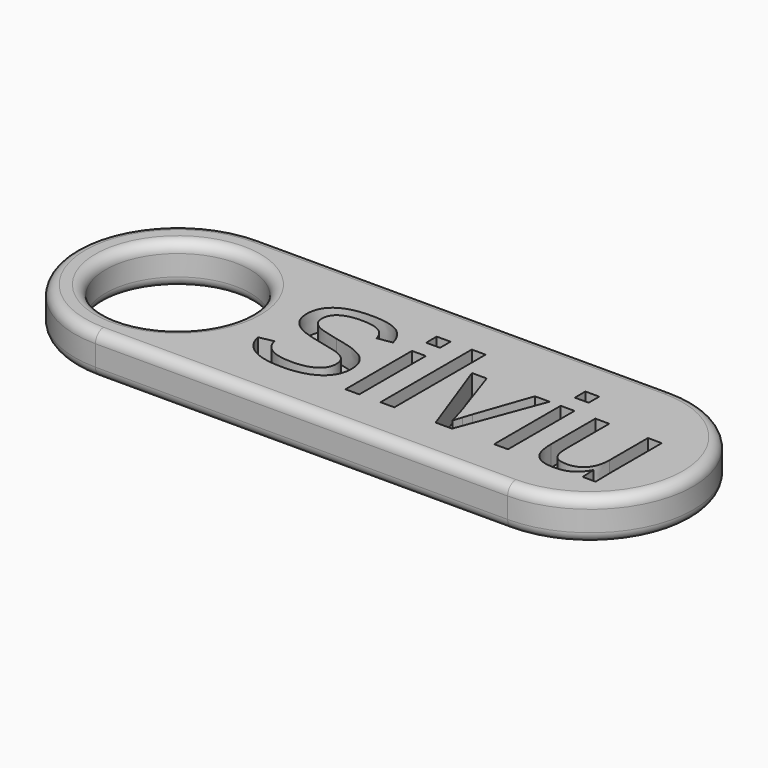
from build123d import *

# Parameters (mm, degrees)
F0_R         = 8.89
F1_DEPTH     = 5.08
F2_TEXT_SIZE = 19.4027777778
F3_DEPTH     = 2.54
F4_R         = 1.27


# Not quite as in the source:
# - Text() gives the source's letters only with a copy of the font that has no kerning and outlines rounded to 1/6400 em; it was checked with that copy


with BuildPart() as f1:
    # F0 (on Top) → F1 (new body)
    with BuildSketch(Plane.XY):
        with BuildLine():
            Line((-25.4, -12.7), (25.4, -12.7))
            ThreePointArc((25.4, -12.7), (38.1, 0), (25.4, 12.7))
            Line((25.4, 12.7), (-25.4, 12.7))
            ThreePointArc((-25.4, 12.7), (-38.1, 0), (-25.4, -12.7))
        make_face()
        with Locations((-25.4, 0)):
            Circle(F0_R, mode=Mode.SUBTRACT)
    extrude(amount=F1_DEPTH)

    # F2 (on face) → F3 (cut)
    with BuildSketch(Plane.XY.offset(5.08)):
        with Locations((-13.4041775174, -6.985)):
            Text('Silviu', F2_TEXT_SIZE, font='Arimo', text_align=(TextAlign.LEFT, TextAlign.BOTTOM))
    extrude(amount=-F3_DEPTH, mode=Mode.SUBTRACT)

    # F4
    f4_edges = [f1.edges().sort_by_distance(p)[0] for p in [
        (-38.1, 0, 5.08),
        (0, -12.7, 0),
        (38.1, 0, 0),
        (0, 12.7, 0),
        (-38.1, 0, 0),
        (-34.29, 0, 0),
        (-34.29, 0, 5.08),
    ]]
    fillet(f4_edges, radius=F4_R)


solid = f1.part
